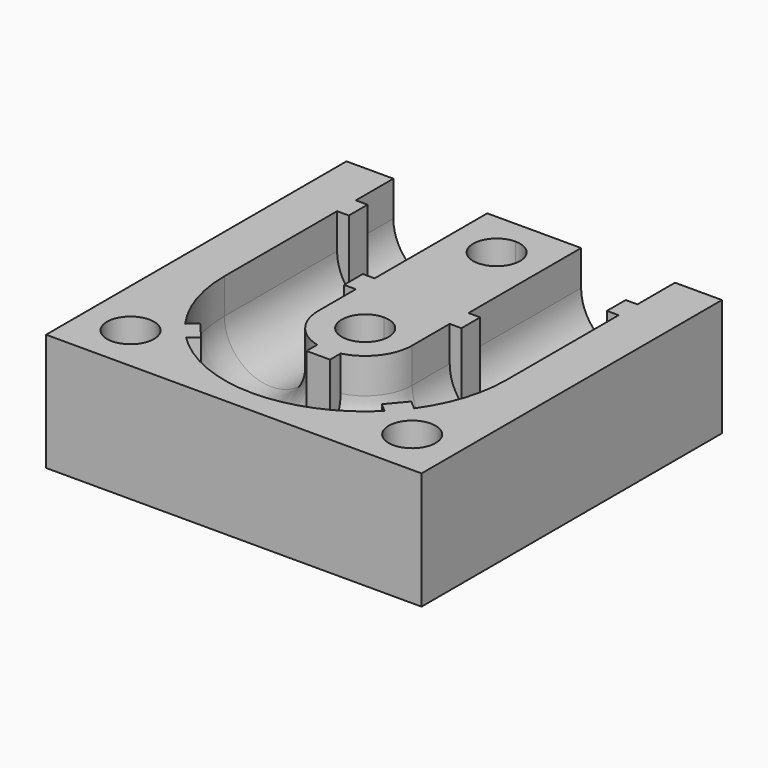
from build123d import *

# Parameters (mm, degrees)
F0_W      = 16
F0_H      = 16
F1_DEPTH  = 5
F2_W      = 2
F2_H      = 9
F3_DEPTH  = 1.5
F4_W      = 2
F4_H      = 9
F8_W      = 0.5
F8_H      = 1
F8_H_2    = 0.5
F9_DEPTH  = 5
F10_R     = 1
F11_DEPTH = 25


# Not quite as in the source:
# - a feature names something its author has since deleted; it is built from what else it names


with BuildPart() as f1:
    # F0 (on Top) → F1 (new body)
    with BuildSketch(Plane.XY):
        with Locations((-8, 8)):
            Rectangle(F0_W, F0_H)
    extrude(amount=F1_DEPTH)

    # F2 (on face) → F3 (cut)
    with BuildSketch(Plane.XY.offset(5)):
        with Locations((-13, 11.5)):
            Rectangle(F2_W, F2_H)
        with BuildLine():
            Line((-12, 7), (-14, 7))
            ThreePointArc((-14, 7), (-8, 1), (-2, 7))
            Line((-2, 7), (-4, 7))
            ThreePointArc((-4, 7), (-8, 3), (-12, 7))
        make_face()
        with BuildLine():
            Line((-10, 16), (-12, 16))
            Line((-12, 16), (-12, 7))
            ThreePointArc((-12, 7), (-8, 3), (-4, 7))
            Line((-4, 7), (-4, 16))
            Line((-4, 16), (-6, 16))
            Line((-6, 16), (-6, 7))
            ThreePointArc((-6, 7), (-8, 5), (-10, 7))
            Line((-10, 7), (-10, 16))
        make_face()
        with Locations((-3, 11.5)):
            Rectangle(F2_W, F2_H)
    extrude(amount=-F3_DEPTH, mode=Mode.SUBTRACT)

    # F4 (on face) → F5 (revolve, cut)
    with BuildSketch(Plane.XY.offset(3.5)):
        with Locations((-13, 11.5)):
            Rectangle(F4_W, F4_H)
    revolve(axis=Axis((-12, 11.5, 3.5), (0, -1, 0)), mode=Mode.SUBTRACT)

    # F6: sweep along a path in F6_path
    with BuildLine(Plane(origin=(-10, 7, 3.5), x_dir=(0, -1, 0), z_dir=(0, 0, -1))) as f6_path:
        ThreePointArc((0, 0), (2, -2), (0, -4))
    # F5_face (on face) → F6 (sweep, cut)
    with BuildSketch(Plane(origin=(-12, 7, 2.6511736368), x_dir=(-1, 0, 0), z_dir=(0, 1, 0))):
        with BuildLine():
            Line((2, 0.8488263632), (-2, 0.8488263632))
            ThreePointArc((-2, 0.8488263632), (0, -1.1511736368), (2, 0.8488263632))
        make_face()
    sweep(path=f6_path.line, mode=Mode.SUBTRACT)

    # F4 (on face) → F7 (revolve, cut)
    with BuildSketch(Plane.XY.offset(3.5)):
        with Locations((-3, 11.5)):
            Rectangle(F4_W, F4_H)
    revolve(axis=Axis((-4, 11.5, 3.5), (0, -1, 0)), mode=Mode.SUBTRACT)

    # F8 (on face) → F9 (join)
    with BuildSketch(Plane.XY.offset(5)):
        with Locations((-13.75, 13.5)):
            Rectangle(F8_W, F8_H)
        with Locations((-10.25, 9.5)):
            Rectangle(F8_W, F8_H)
        with Locations((-5.75, 9.5)):
            Rectangle(F8_W, F8_H)
        with Locations((-2.25, 13.5)):
            Rectangle(F8_W, F8_H)
        with BuildLine():
            Line((-12.4976444751, 3.8310784478), (-12.8785175711, 3.5071406687))
            ThreePointArc((-12.8785175711, 3.5071406687), (-12.570477152, 3.1127466505), (-12.2306420128, 2.7453944767))
            Line((-12.2306420128, 2.7453944767), (-11.8497689168, 3.0693322558))
            Line((-11.8497689168, 3.0693322558), (-12.4976444751, 3.8310784478))
        make_face()
        with BuildLine():
            ThreePointArc((-3.7693579872, 2.7453944767), (-3.429522848, 3.1127466505), (-3.1214824289, 3.5071406687))
            Line((-3.1214824289, 3.5071406687), (-3.5023555249, 3.8310784478))
            Line((-3.5023555249, 3.8310784478), (-4.1502310832, 3.0693322558))
            Line((-4.1502310832, 3.0693322558), (-3.7693579872, 2.7453944767))
        make_face()
        with Locations((-8.25, 4.75)):
            Rectangle(F8_W, F8_H_2)
        with Locations((-7.75, 4.75)):
            Rectangle(F8_W, F8_H_2)
        with Locations((-8.25, 5.25)):
            Rectangle(F8_W, F8_H_2)
        with Locations((-7.75, 5.25)):
            Rectangle(F8_W, F8_H_2)
    extrude(amount=-F9_DEPTH)

    # F10 (on face) → F11 (cut)
    with BuildSketch(Plane.XY.offset(5)):
        with BuildLine():
            ThreePointArc((-7, 14), (-7.2928932188, 14.7071067812), (-8, 15))
            Line((-8, 15), (-8, 13))
            ThreePointArc((-8, 13), (-7.2928932188, 13.2928932188), (-7, 14))
        make_face()
        with BuildLine():
            Line((-8, 13), (-8, 15))
            ThreePointArc((-8, 15), (-9, 14), (-8, 13))
        make_face()
        with BuildLine():
            Line((-8, 8), (-8, 6))
            ThreePointArc((-8, 6), (-7.2928932188, 6.2928932188), (-7, 7))
            ThreePointArc((-7, 7), (-7.2928932188, 7.7071067812), (-8, 8))
        make_face()
        with BuildLine():
            ThreePointArc((-8, 8), (-9, 7), (-8, 6))
            Line((-8, 6), (-8, 8))
        make_face()
        with Locations((-14, 2)):
            Circle(F10_R)
        with Locations((-2, 2)):
            Circle(F10_R)
    extrude(amount=-F11_DEPTH, mode=Mode.SUBTRACT)


solid = f1.part
